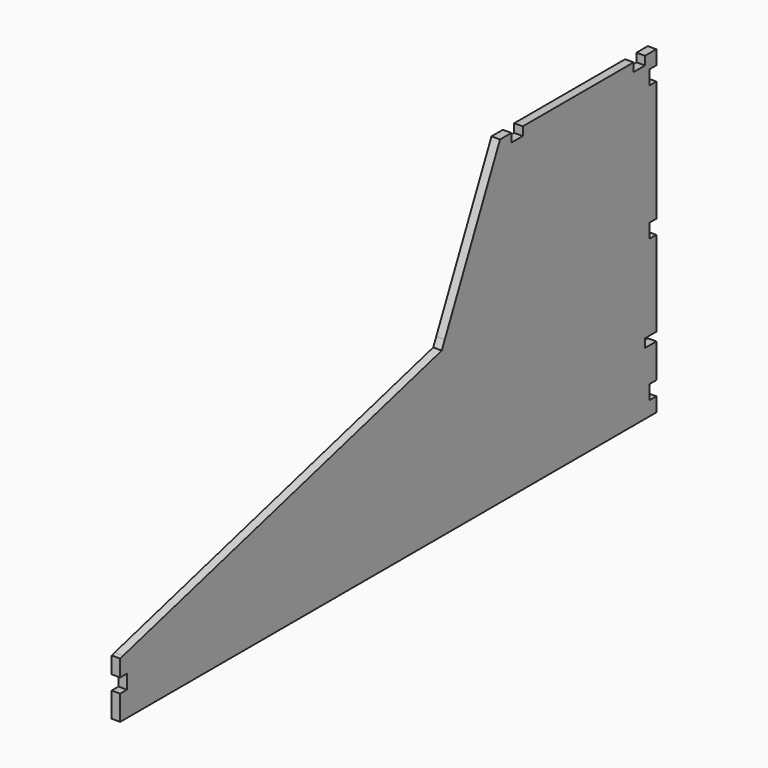
from build123d import *

# Parameters (mm, degrees)
F0_W      = 200
F0_H      = 460
F1_DEPTH  = 12
F2_W      = 12
F2_H      = 20
F2_W_2    = 20
F2_H_2    = 22
F3_DEPTH  = 25
F4_DEPTH  = 10
F6_W      = 12
F6_H      = 20
F7_DEPTH  = 12
F8_W      = 20
F8_H      = 12
F9_DEPTH  = 25
F11_DEPTH = 25
F12_W     = 5.3429044291
F12_H     = 20
F12_H_2   = 35
F13_DEPTH = 12


# Not quite as in the source:
# - a feature of the source that left no trace in its solid (it failed there, or was rolled back) is left out
# - a feature names something its author has since deleted; it is built from what else it names


with BuildPart() as f1:
    # F0 (on Right) → F1 (new body)
    with BuildSketch(Plane.YZ):
        Polygon((-738, 0), (0, 0), (0, 460), (-70.3818810435, 460), (-172.2238128496, 241.5992724437), (-738, 90), align=None)
        with Locations((100, 230)):
            Rectangle(F0_W, F0_H)
    extrude(amount=F1_DEPTH)

    # F2 (on face) → F3 (cut)
    with BuildSketch(Plane.YZ.offset(12)):
        with Locations((194, 30)):
            Rectangle(F2_W, F2_H)
        with Locations((194, 230)):
            Rectangle(F2_W, F2_H)
        with Locations((194, 420)):
            Rectangle(F2_W, F2_H)
        with Locations((170, 449)):
            Rectangle(F2_W_2, F2_H_2)
        Polygon((-35.0449576251, 460), (-55.0449576251, 460), (-55.0449576251, 450), (-55.0449576251, 438), (-35.0449576251, 438), align=None)
    extrude(amount=-F3_DEPTH, mode=Mode.SUBTRACT)

    # F4 (cut): faces of the model
    f4_faces = [f1.faces().sort_by_distance(p)[0] for p in [
        (6, -62.7134193343, 460),
        (6, 62.4775211875, 460),
        (6, 190, 460),
    ]]
    extrude(f4_faces, amount=-F4_DEPTH, mode=Mode.SUBTRACT)

    # F6 (on face) → F7 (cut)
    with BuildSketch(Plane.XZ.offset(738)):
        with Locations((6, 45)):
            Rectangle(F6_W, F6_H)
    extrude(amount=-F7_DEPTH, mode=Mode.SUBTRACT)

    # F8 (on face) → F9 (cut)
    with BuildSketch(Plane.YZ.offset(12)):
        with Locations((190, 94)):
            Rectangle(F8_W, F8_H)
        Polygon((-70.3818810435, 460), (-75.0449576251, 450), (-70.3818810435, 450), align=None)
    extrude(amount=-F9_DEPTH, mode=Mode.SUBTRACT)

    # F10 (on face) → F11 (cut)
    with BuildSketch(Plane.YZ.offset(12)):
        Polygon((-177.5667172787, 230.14137692), (-172.2238128496, 241.5992724437), (-738, 90), (-738, 79.9737314033), align=None)
    extrude(amount=-F11_DEPTH, mode=Mode.SUBTRACT)

    # F12 (on face) → F13 (join)
    with BuildSketch(Plane.YZ.offset(12)):
        Polygon((-738, 55), (-738, 79.9737314033), (-743.3429044291, 78.5421044763), (-743.3429044291, 55), align=None)
        with Locations((-728.6714522145, 45)):
            Rectangle(F12_W, F12_H)
        with Locations((-740.6714522145, 17.5)):
            Rectangle(F12_W, F12_H_2)
    extrude(amount=-F13_DEPTH)


solid = f1.part
